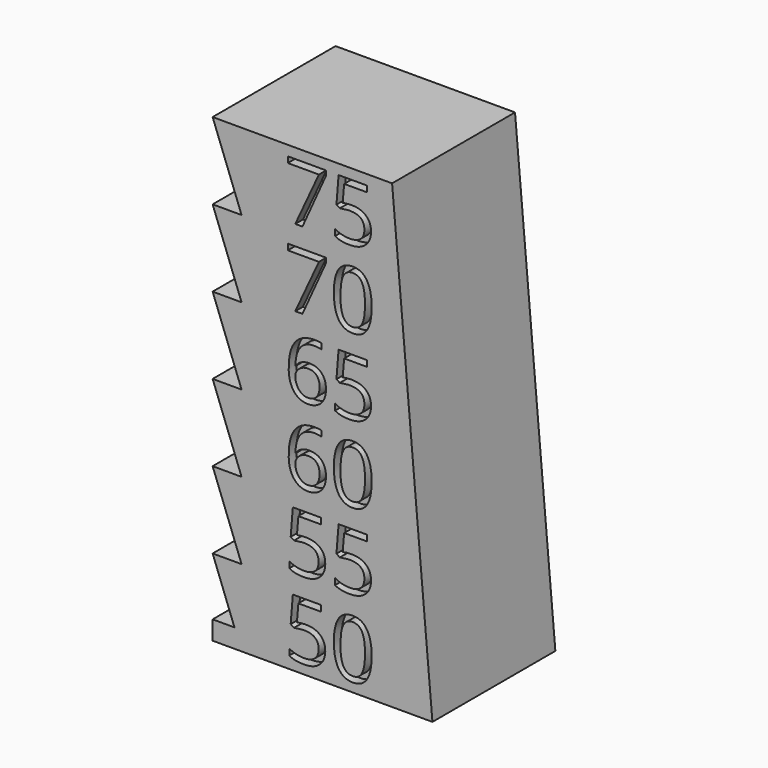
from build123d import *

# Parameters (mm, degrees)
F1_DEPTH     = 12.7
F2_TEXT_SIZE = 6.6145833333
F3_DEPTH     = 0.79375


# Not quite as in the source:
# - ends of sketch curves that miss each other by under 0.0002 mm in the source are joined
# - Text() gives the source's letters only with a copy of the font that has no kerning and outlines rounded to 1/6400 em; it was checked with that copy


with BuildPart() as f1:
    # F0 (on Front) → F1 (new body)
    with BuildSketch(Plane.XZ):
        Polygon((5.4643177427, 0), (2.1309996624, 38.1), (-12.7, 38.1), (-10.3094507526, 31.7500010133), (-12.7, 31.7500010133), (-10.3094502555, 25.399999693), (-12.7, 25.399999693), (-10.3094504597, 19.0500002354), (-12.7, 19.0500002354), (-10.3094503133, 12.6999998465), (-12.7, 12.6999998465), (-10.3094503422, 6.3499999233), (-12.7, 6.3499999233), (-10.8951350373, 1.55575), (-12.7, 1.55575), (-12.7, 0), align=None)
    extrude(amount=F1_DEPTH)

    # F2 (on face) → F3 (cut)
    with BuildSketch(Plane.XZ.offset(12.7)):
        with Locations((-6.7928411286, 32.54375)):
            Text('75', F2_TEXT_SIZE, font='Open Sans', text_align=(TextAlign.LEFT, TextAlign.BOTTOM))
        with Locations((-6.7928411286, 26.19375)):
            Text('70', F2_TEXT_SIZE, font='Open Sans', text_align=(TextAlign.LEFT, TextAlign.BOTTOM))
        with Locations((-6.7928411286, 19.84375)):
            Text('65', F2_TEXT_SIZE, font='Open Sans', text_align=(TextAlign.LEFT, TextAlign.BOTTOM))
        with Locations((-6.7928411286, 13.49375)):
            Text('60', F2_TEXT_SIZE, font='Open Sans', text_align=(TextAlign.LEFT, TextAlign.BOTTOM))
        with Locations((-6.7928411286, 7.14375)):
            Text('55', F2_TEXT_SIZE, font='Open Sans', text_align=(TextAlign.LEFT, TextAlign.BOTTOM))
        with Locations((-6.7928411286, 0.79375)):
            Text('50', F2_TEXT_SIZE, font='Open Sans', text_align=(TextAlign.LEFT, TextAlign.BOTTOM))
    extrude(amount=-F3_DEPTH, mode=Mode.SUBTRACT)


solid = f1.part
